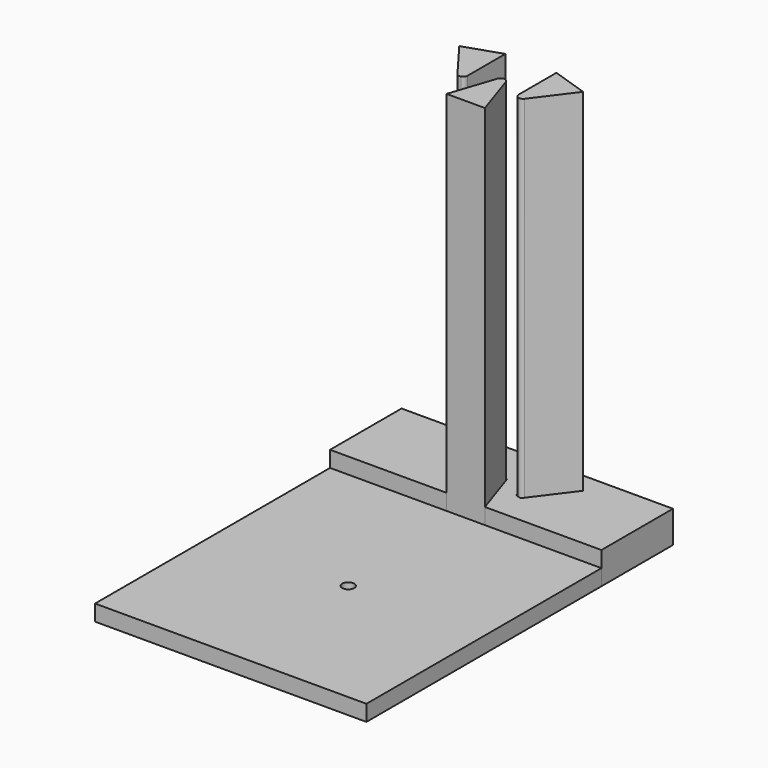
from build123d import *

# Parameters (mm, degrees)
F1_DEPTH      = 152.4
F0_R          = 2.38125
F2_DEPTH      = 6.35
F3_DEPTH      = 12.7
F4_T1_DEPTH   = 158.8075491552
F4_2_T1_DEPTH = 158.8075494663
F4_3_T1_DEPTH = 158.8075494663


# Not quite as in the source:
# - a fillet or chamfer that OpenCascade refuses, or shapes differently, is made with other operations: its cross-section is extruded or revolved along the edge and cut away or added


with BuildPart() as f1:
    # F0 (on Top) → F1 (new body)
    with BuildSketch(Plane.XY):
        Polygon((-10.16, 70.724540249), (-10.16, 90.805), (-24.6179332403, 85.98568818), (-12.56965591, 69.921321489), align=None)
    extrude(amount=F1_DEPTH)

    # F4: fillet of radius 1.778 on 2 edges, made by hand

    # F4_s2 → F4_t1 (cut)
    with BuildSketch(Plane.XY.offset(-3.2037745776)):
        with BuildLine():
            ThreePointArc((-11.3757469543, 70.319291202), (-10.4956113708, 70.9664352271), (-10.16, 72.0060500801))
            Line((-10.16, 72.0060500801), (-10.16, 70.724540249))
            Line((-10.16, 70.724540249), (-11.3757469543, 70.319291202))
        make_face()
        with BuildLine():
            ThreePointArc((-13.3385619031, 70.946529283), (-12.4463038366, 70.3162043054), (-11.3539089557, 70.326570536))
            Line((-11.3539089557, 70.326570536), (-12.56965591, 69.921321489))
            Line((-12.56965591, 69.921321489), (-13.3385619031, 70.946529283))
        make_face()
    extrude(amount=F4_T1_DEPTH, mode=Mode.SUBTRACT)


with BuildPart() as f1b:
    # F0 (on Top) → F1, piece 2 (new body)
    with BuildSketch(Plane.XY):
        Polygon((24.6179334623, 85.9856888459), (10.16, 90.805), (10.16, 70.7245368579), (12.569655577, 69.9213183322), align=None)
    extrude(amount=F1_DEPTH)

    # F4#2: fillet of radius 1.778 on 2 edges, made by hand

    # F4_2_s2 → F4_2_t1 (cut)
    with BuildSketch(Plane.XY.offset(-3.2037747331)):
        with BuildLine():
            ThreePointArc((10.16, 72.0060467512), (10.4956113948, 70.9664318651), (11.375747032, 70.3192878473))
            Line((11.375747032, 70.3192878473), (10.16, 70.7245368579))
            Line((10.16, 70.7245368579), (10.16, 72.0060467512))
        make_face()
        with BuildLine():
            ThreePointArc((11.353908545, 70.3265673429), (12.4463034655, 70.3162011748), (13.338561513, 70.9465262469))
            Line((13.338561513, 70.9465262469), (12.569655577, 69.9213183322))
            Line((12.569655577, 69.9213183322), (11.353908545, 70.3265673429))
        make_face()
    extrude(amount=F4_2_T1_DEPTH, mode=Mode.SUBTRACT)


with BuildPart() as f1c:
    # F0 (on Top) → F1, piece 3 (new body)
    with BuildSketch(Plane.XY):
        Polygon((0, 77.47), (0, 58.42), (7.62, 58.42), (1.27, 77.47), align=None)
        Polygon((-1.27, 77.47), (-7.62, 58.42), (0, 58.42), (0, 77.47), align=None)
    extrude(amount=F1_DEPTH)

    # F4#3: fillet of radius 1.778 on 2 edges, made by hand

    # F4_3_s2 → F4_3_t1 (cut)
    with BuildSketch(Plane.XY.offset(-3.2037747331)):
        with BuildLine():
            ThreePointArc((0.0115098933, 77.47), (-1.0281049929, 77.1343886052), (-1.6752490107, 76.254252968))
            Line((-1.6752490107, 76.254252968), (-1.27, 77.47))
            Line((-1.27, 77.47), (0.0115098933, 77.47))
        make_face()
        with BuildLine():
            ThreePointArc((1.6752490107, 76.254252968), (1.0281049929, 77.1343886052), (-0.0115098933, 77.47))
            Line((-0.0115098933, 77.47), (1.27, 77.47))
            Line((1.27, 77.47), (1.6752490107, 76.254252968))
        make_face()
    extrude(amount=F4_3_T1_DEPTH, mode=Mode.SUBTRACT)


with BuildPart() as f2:
    # F0 (on Top) → F2 (new body)
    with BuildSketch(Plane.XY):
        Polygon((-7.62, 58.42), (-53.975, 58.42), (-53.975, -58.42), (53.975, -58.42), (53.975, 58.42), (7.62, 58.42), (0, 58.42), align=None)
        Circle(F0_R, mode=Mode.SUBTRACT)
    extrude(amount=F2_DEPTH)


with BuildPart() as f3:
    # F0 (on Top) → F3 (new body)
    with BuildSketch(Plane.XY):
        Polygon((-53.975, 90.805), (-53.975, 58.42), (-7.62, 58.42), (-1.27, 77.47), (0, 77.47), (0, 90.805), (-10.16, 90.805), align=None)
        Polygon((-24.6179332403, 85.98568818), (-10.16, 90.805), (-10.16, 70.724540249), (-12.56965591, 69.921321489), align=None, mode=Mode.SUBTRACT)
        Polygon((1.27, 77.47), (7.62, 58.42), (53.975, 58.42), (53.975, 90.805), (10.16, 90.805), (0, 90.805), (0, 77.47), align=None)
        Polygon((10.16, 70.7245368579), (10.16, 90.805), (24.6179334623, 85.9856888459), (12.569655577, 69.9213183322), align=None, mode=Mode.SUBTRACT)
        Polygon((53.975, 93.98), (0, 93.98), (0, 90.805), (10.16, 90.805), (53.975, 90.805), align=None)
        Polygon((-53.975, 93.98), (-53.975, 90.805), (-10.16, 90.805), (0, 90.805), (0, 93.98), align=None)
    extrude(amount=F3_DEPTH)


solid = Compound([f1.part, f1b.part, f1c.part, f2.part, f3.part])
